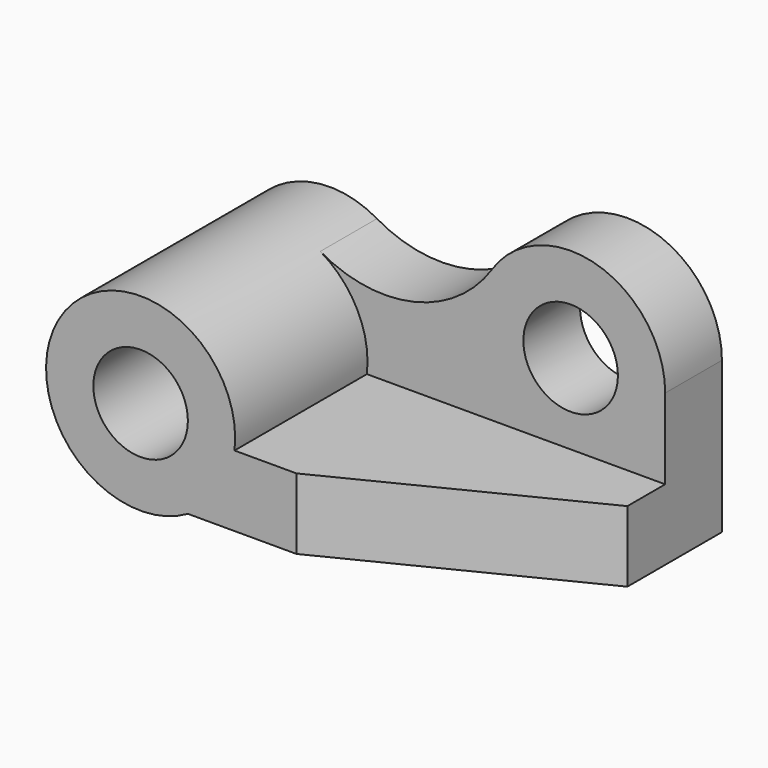
from build123d import *
from build123d import SkipClean  # not in build123d's __all__

# Parameters (mm, degrees)
F0_R     = 10
F1_DEPTH = 15
F2_R     = 10
F3_DEPTH = 35
F5_DEPTH = 35
F7_DEPTH = 15


# Not quite as in the source:
# - after a boolean that leaves OpenCascade's solid faulty, fix() repairs it


with BuildPart() as f1:
    # F0 (on Front) → F1 (new body)
    with BuildSketch(Plane.XZ):
        with BuildLine():
            ThreePointArc((46.3350602938, 25.7917141365), (29.8412578998, 14.3770862565), (10, 17.3205080757))
            ThreePointArc((10, 17.3205080757), (-20, 0), (10, -17.3205080757))
            Line((10, -17.3205080757), (82.9639062402, -17.3205080757))
            Line((82.9639062402, -17.3205080757), (82.9639062402, 14.6794919243))
            ThreePointArc((82.9639062402, 14.6794919243), (68.7700702523, 33.818155918), (46.3350602938, 25.7917141365))
        make_face()
        with BuildLine():
            ThreePointArc((5, 8.6602540378), (8.6602540378, 5), (10, 0))
            ThreePointArc((10, 0), (-8.6602540378, -5), (5, 8.6602540378))
        make_face(mode=Mode.SUBTRACT)
        with Locations((62.9639062402, 14.6794919243)):
            Circle(F0_R, mode=Mode.SUBTRACT)
    extrude(amount=F1_DEPTH)

    # F2 (on face) → F3 (join)
    with BuildSketch(Plane.XZ.offset(15)):
        with BuildLine():
            ThreePointArc((10, -17.3205080757), (17.3205080757, -10), (20, 0))
            ThreePointArc((20, 0), (17.3205080757, 10), (10, 17.3205080757))
            ThreePointArc((10, 17.3205080757), (-20, 0), (10, -17.3205080757))
        make_face()
        Circle(F2_R, mode=Mode.SUBTRACT)
    with SkipClean():  # cleaning this boolean's faces spoils the solid; the shape is the same uncleaned
        extrude(amount=F3_DEPTH)

    # F4 (on face) → F5 (join)
    with BuildSketch(Plane.XZ.offset(15)):
        with BuildLine():
            Line((10, -17.3205080757), (82.9639062402, -17.3205080757))
            Line((82.9639062402, -17.3205080757), (82.9639062402, -2.3205080757))
            Line((82.9639062402, -2.3205080757), (19.8649249249, -2.3205080757))
            ThreePointArc((19.8649249249, -2.3205080757), (16.710129718, -10.9896116769), (10, -17.3205080757))
        make_face()
    extrude(amount=F5_DEPTH)

    add(f1.part.fix(), mode=Mode.REPLACE)

    # F6 (on face) → F7 (cut, through all)
    with BuildSketch(Plane.XY.offset(-2.3205080757)):
        Polygon((82.9639062402, -50), (82.9639062402, -25), (32.9639062402, -50), align=None)
    extrude(amount=-F7_DEPTH, mode=Mode.SUBTRACT)


solid = f1.part
